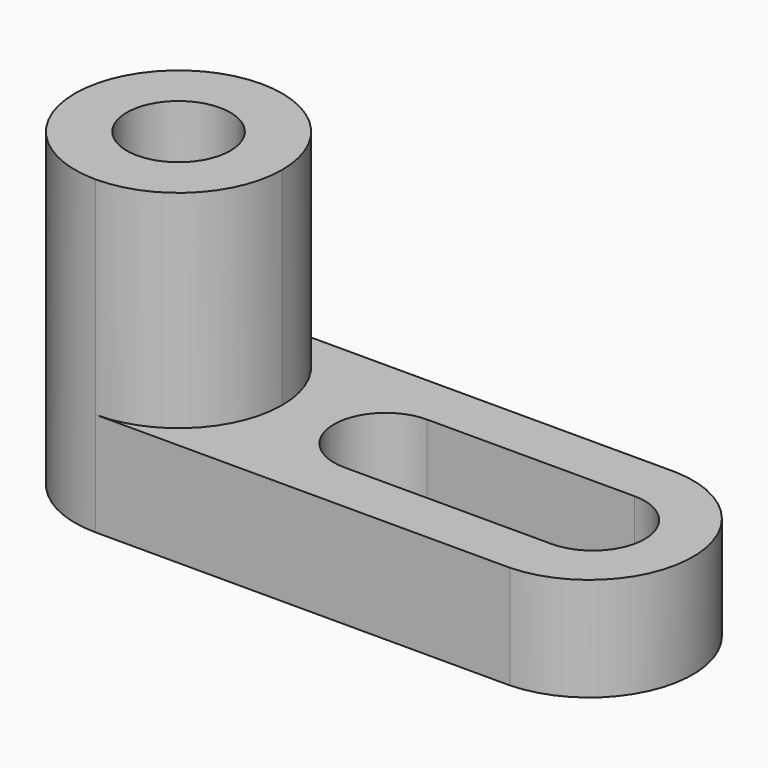
from build123d import *

# Parameters (mm, degrees)
F1_DEPTH = 25.4
F3_DEPTH = 12.701
F5_DEPTH = 38.101
F7_DEPTH = 25.4


with BuildPart() as f1:
    # F0 (on Front) → F1 (new body)
    with BuildSketch(Plane.XZ):
        Polygon((0, 38.1), (0, 0), (76.2, 0), (76.2, 12.7), (25.4, 12.7), (25.4, 38.1), align=None)
    extrude(amount=F1_DEPTH)

    # F2 (on face) → F3 (cut, through all)
    with BuildSketch(Plane.XY.offset(12.7)):
        with BuildLine():
            Line((76.2, 0), (63.5, 0))
            ThreePointArc((63.5, 0), (75.756906611, -12.7), (63.5, -25.4))
            Line((63.5, -25.4), (76.2, -25.4))
            Line((76.2, -25.4), (76.2, 0))
        make_face()
        with BuildLine():
            ThreePointArc((69.85, -12.7), (67.9901280605, -8.2098719395), (63.5, -6.35))
            Line((63.5, -6.35), (63.5, -19.05))
            ThreePointArc((63.5, -19.05), (67.9901280605, -17.1901280605), (69.85, -12.7))
        make_face()
        with BuildLine():
            Line((63.5, -19.05), (63.5, -6.35))
            ThreePointArc((63.5, -6.35), (57.15, -12.7), (63.5, -19.05))
        make_face()
        with BuildLine():
            ThreePointArc((63.5, -19.05), (57.15, -12.7), (63.5, -6.35))
            Line((63.5, -6.35), (38.1, -6.35))
            ThreePointArc((38.1, -6.35), (42.5901280605, -8.2098719395), (44.45, -12.7))
            ThreePointArc((44.45, -12.7), (42.5901280605, -17.1901280605), (38.1, -19.05))
            Line((38.1, -19.05), (63.5, -19.05))
        make_face()
        with BuildLine():
            Line((38.1, -19.05), (38.1, -6.35))
            ThreePointArc((38.1, -6.35), (31.75, -12.7), (38.1, -19.05))
        make_face()
        with BuildLine():
            ThreePointArc((44.45, -12.7), (42.5901280605, -8.2098719395), (38.1, -6.35))
            Line((38.1, -6.35), (38.1, -19.05))
            ThreePointArc((38.1, -19.05), (42.5901280605, -17.1901280605), (44.45, -12.7))
        make_face()
    extrude(amount=-F3_DEPTH, mode=Mode.SUBTRACT)

    # F4 (on face) → F5 (cut, through all)
    with BuildSketch(Plane.XY.offset(38.1)):
        with BuildLine():
            ThreePointArc((0, -12.7), (3.7197438789, -3.7197438789), (12.7, 0))
            Line((12.7, 0), (0, 0))
            Line((0, 0), (0, -12.7))
        make_face()
        with BuildLine():
            Line((0, -25.4), (12.7, -25.4))
            ThreePointArc((12.7, -25.4), (3.7197438789, -21.6802561211), (0, -12.7))
            Line((0, -12.7), (0, -25.4))
        make_face()
        with BuildLine():
            ThreePointArc((6.35, -12.7), (12.7, -19.05), (19.05, -12.7))
            Line((19.05, -12.7), (6.35, -12.7))
        make_face()
        with BuildLine():
            Line((6.35, -12.7), (19.05, -12.7))
            ThreePointArc((19.05, -12.7), (12.7, -6.35), (6.35, -12.7))
        make_face()
    extrude(amount=-F5_DEPTH, mode=Mode.SUBTRACT)

    # F6 (on face) → F7 (cut)
    with BuildSketch(Plane.XY.offset(38.1)):
        with BuildLine():
            Line((25.4, -25.4), (25.4, -12.7))
            ThreePointArc((25.4, -12.7), (21.6802561211, -21.6802561211), (12.7, -25.4))
            Line((12.7, -25.4), (25.4, -25.4))
        make_face()
        with BuildLine():
            ThreePointArc((12.7, 0), (21.6802561211, -3.7197438789), (25.4, -12.7))
            Line((25.4, -12.7), (25.4, 0))
            Line((25.4, 0), (12.7, 0))
        make_face()
    extrude(amount=-F7_DEPTH, mode=Mode.SUBTRACT)


solid = f1.part
